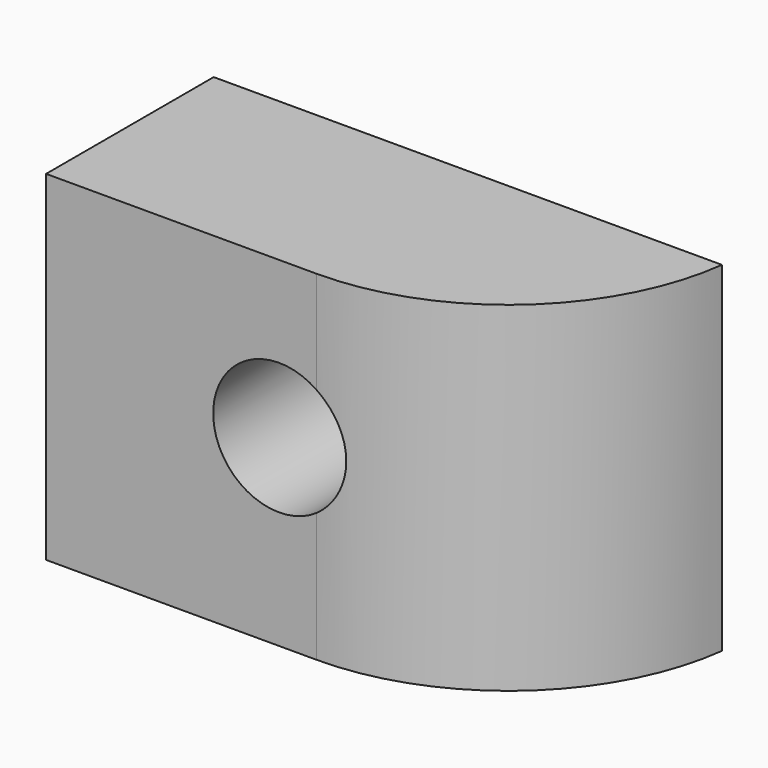
from build123d import *

# Parameters (mm, degrees)
F0_W        = 106.7279540002
F0_H        = 43.9982321113
F1_DEPTH    = 71.374
F2_R        = 13.8308303795
F3_DEPTH    = 43.9982321113
F4_T1_DEPTH = 320.8185282784


# Not quite as in the source:
# - a fillet or chamfer that OpenCascade refuses, or shapes differently, is made with other operations: its cross-section is extruded or revolved along the edge and cut away or added


with BuildPart() as f1:
    # F0 (on Top) → F1 (new body)
    with BuildSketch(Plane.XY):
        with Locations((10.7528511435, 12.0171392336)):
            Rectangle(F0_W, F0_H)
    extrude(amount=F1_DEPTH)

    # F2 (on face) → F3 (cut, through all)
    with BuildSketch(Plane.XZ.offset(9.981976822)):
        with Locations((6.3148764893, 38.5243110359)):
            Circle(F2_R)
    extrude(amount=-F3_DEPTH, mode=Mode.SUBTRACT)

    # F4: fillet of radius 50.2832400771 on 1 edges, made by hand

    # F4_s2 → F4_t1 (cut)
    with BuildSketch(Plane.XY.offset(-124.7222641392)):
        with BuildLine():
            ThreePointArc((64.1168281436, 34.0162552893), (47.4873096457, 2.5889655454), (14.2279224879, -9.981976822))
            Line((14.2279224879, -9.981976822), (64.1168281436, -9.981976822))
            Line((64.1168281436, -9.981976822), (64.1168281436, 34.0162552893))
        make_face()
    extrude(amount=F4_T1_DEPTH, mode=Mode.SUBTRACT)


solid = f1.part
